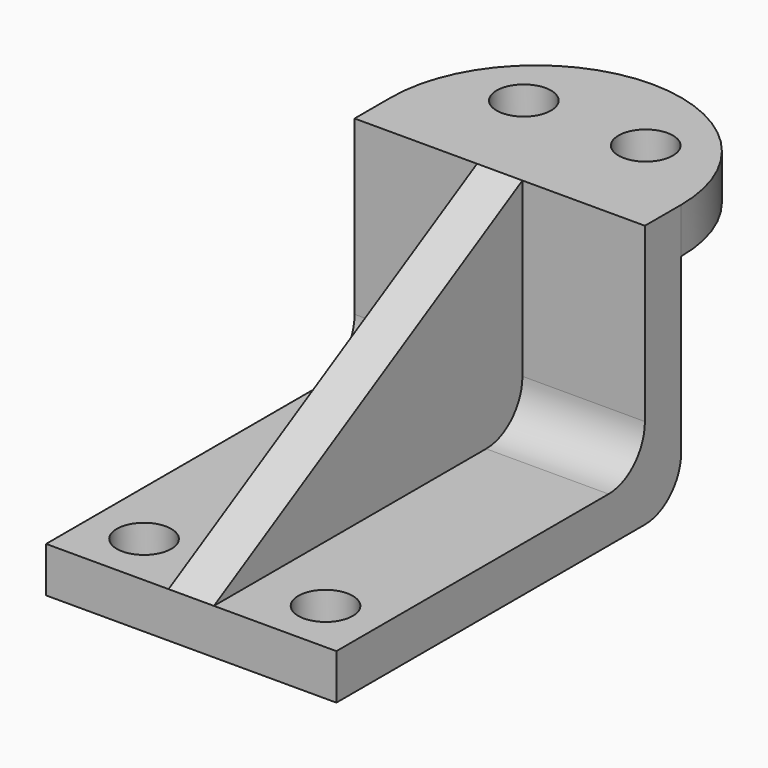
from build123d import *

# Parameters (mm, degrees)
F1_DEPTH = 5
F2_DEPTH = 32
F4_R     = 6
F5_DEPTH = 58.001


with BuildPart() as f1:
    # F0 (on Right) → F1 (new body, symmetric)
    with BuildSketch(Plane.YZ):
        with BuildLine():
            Line((85, 48), (0, 0))
            Line((0, 0), (75, 0))
            ThreePointArc((75, 0), (82.0710678119, 2.9289321881), (85, 10))
            Line((85, 10), (85, 48))
        make_face()
        with BuildLine():
            Line((75, 0), (0, 0))
            Line((0, 0), (0, -10))
            Line((0, -10), (85, -10))
            ThreePointArc((85, -10), (92.0710678119, -7.0710678119), (95, 0))
            Line((95, 0), (95, 38))
            Line((95, 38), (127, 38))
            Line((127, 38), (127, 48))
            Line((127, 48), (85, 48))
            Line((85, 48), (85, 10))
            ThreePointArc((85, 10), (82.0710678119, 2.9289321881), (75, 0))
        make_face()
    extrude(amount=F1_DEPTH, both=True)

    # F0 (on Right) → F2 (join, symmetric)
    with BuildSketch(Plane.YZ):
        with BuildLine():
            Line((75, 0), (0, 0))
            Line((0, 0), (0, -10))
            Line((0, -10), (85, -10))
            ThreePointArc((85, -10), (92.0710678119, -7.0710678119), (95, 0))
            Line((95, 0), (95, 38))
            Line((95, 38), (127, 38))
            Line((127, 38), (127, 48))
            Line((127, 48), (85, 48))
            Line((85, 48), (85, 10))
            ThreePointArc((85, 10), (82.0710678119, 2.9289321881), (75, 0))
        make_face()
    extrude(amount=F2_DEPTH, both=True)

    # F4 (on face) → F5 (cut, through all)
    with BuildSketch(Plane.XY.offset(48)):
        with BuildLine():
            ThreePointArc((-32, 95), (-22.6274171136, 117.6274168823), (-3.272e-07, 127))
            Line((-3.272e-07, 127), (-32, 127))
            Line((-32, 127), (-32, 95))
        make_face()
        with BuildLine():
            ThreePointArc((-3.272e-07, 127), (22.6274168823, 117.6274171136), (32, 95))
            Line((32, 95), (32, 127))
            Line((32, 127), (-3.272e-07, 127))
        make_face()
        with Locations((13.4350288425, 108.4350288425)):
            Circle(F4_R)
        with Locations((-13.4350288425, 108.4350288425)):
            Circle(F4_R)
        with Locations((-20, 12)):
            Circle(F4_R)
        with Locations((20, 12)):
            Circle(F4_R)
    extrude(amount=-F5_DEPTH, mode=Mode.SUBTRACT)


solid = f1.part
